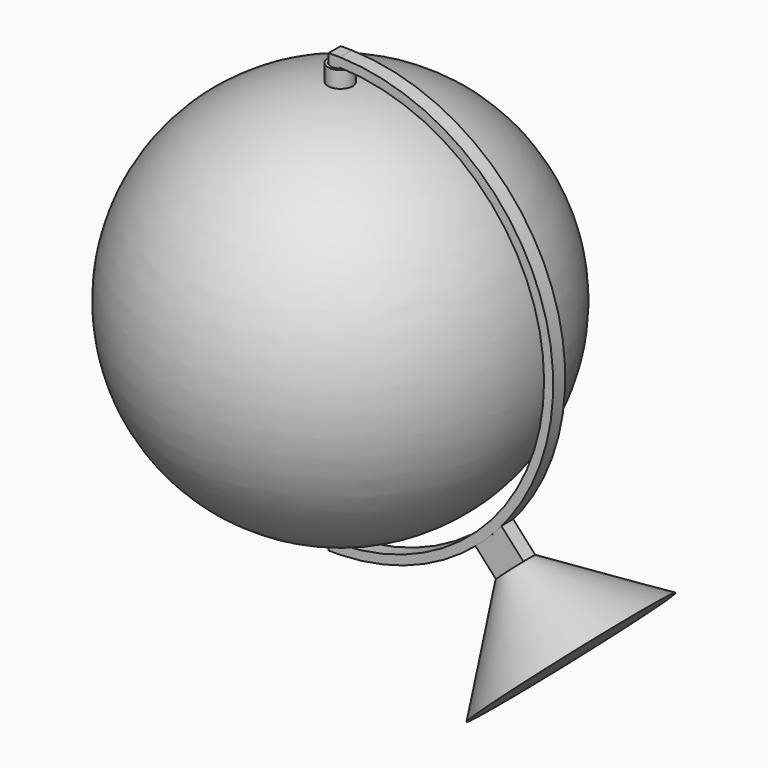
from build123d import *

# Parameters (mm, degrees)
F2_R          = 2.5272068821
F2_R_2        = 1.9710754147
F3_DEPTH      = 37.846
F3_DEPTH_BACK = 47.244
F5_DEPTH      = 1.524
F5_DEPTH_BACK = 1.5494
F9_DEPTH      = 1.4732
F9_DEPTH_BACK = 1.5494


with BuildPart() as f1:
    # F0 (on Front) → F1 (revolve)
    with BuildSketch(Plane.XZ):
        with BuildLine():
            ThreePointArc((0, -44.4500036538), (39.6567446185, -4.9550831318), (0, 34.5398373902))
            Line((0, 34.5398373902), (0, -44.4500036538))
        make_face()
    revolve(axis=Axis((0, 0, -4.9550831318), (0, 0, -1)))


with BuildPart() as f3:
    # F2 (on Top) → F3 (new body, two sides)
    with BuildSketch(Plane.XY) as f3_sk:
        Circle(F2_R)
        Circle(F2_R_2, mode=Mode.SUBTRACT)
    extrude(amount=F3_DEPTH)
    extrude(f3_sk.sketch, amount=-F3_DEPTH_BACK)


with BuildPart() as f5:
    # F4 (on Front) → F5 (new body, two sides)
    with BuildSketch(Plane.XZ) as f5_sk:
        Polygon((1.1481613619, 39.8442782462), (-1.1786745163, 39.8442782462), (-1.1786745163, 35.0171774626), (1.1481613619, 35.0171774626), (1.1481613619, 37.9777580962), align=None)
        with BuildLine():
            ThreePointArc((1.1481613619, -49.8090833426), (44.7845028948, -4.9824025482), (1.1481613619, 39.8442782462))
            Line((1.1481613619, 39.8442782462), (1.1481613619, 37.9777580962))
            ThreePointArc((1.1481613619, 37.9777580962), (42.9186878637, -4.9824025482), (1.1481613619, -47.9425631926))
            Line((1.1481613619, -47.9425631926), (1.1481613619, -49.8090833426))
        make_face()
        Polygon((-1.1786745163, -49.8090833426), (1.1481613619, -49.8090833426), (1.1481613619, -47.9425631926), (1.1481613619, -44.8573455215), (-1.1786745163, -44.8573455215), align=None)
    extrude(amount=F5_DEPTH)
    extrude(f5_sk.sketch, amount=-F5_DEPTH_BACK)


with BuildPart() as f7:
    # F6 (on Front) → F7 (revolve)
    with BuildSketch(Plane.XZ):
        Polygon((38.6343021336, -38.8564354593), (35.8513659946, -41.385093744), (47.2318957666, -53.9100314847), (61.7852827642, -40.6863925782), align=None)
    revolve(axis=Axis((41.5416308806, 0, -47.6475626144), (0.672485861, 0, -0.7401099693)))


with BuildPart() as f9:
    # F6 (on Front) → F9 (new body, two sides)
    with BuildSketch(Plane.XZ) as f9_sk:
        Polygon((34.1358935437, -33.905674058), (28.5700212656, -38.9629906275), (33.0684298556, -43.9137520288), (35.8513659946, -41.385093744), (38.6343021336, -38.8564354593), align=None)
    extrude(amount=F9_DEPTH)
    extrude(f9_sk.sketch, amount=-F9_DEPTH_BACK)


solid = Compound([f1.part, f3.part, f5.part, f7.part, f9.part])
